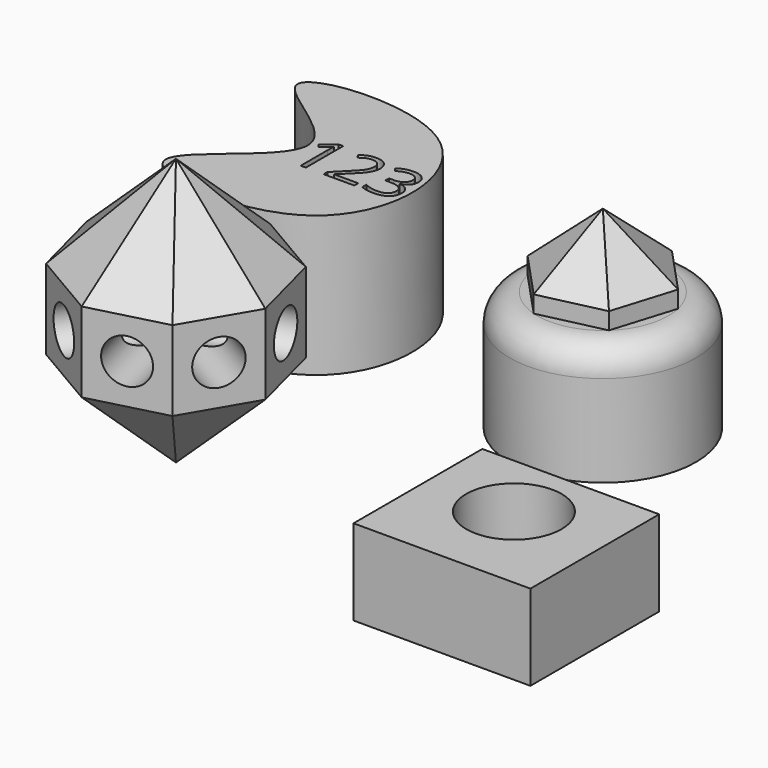
from build123d import *

# Parameters (mm, degrees)
F0_R          = 53.2418373221
F1_DEPTH      = 68.326
F2_R          = 15.9434663659
F3_W          = 92.0383110642
F3_H          = 48.9154662937
F4_DEPTH      = 101.092
F5_R          = 27.2499431861
F6_DEPTH      = 168.402
F8_DEPTH      = 102.87
F9_DEPTH      = 41.91
F11_DEPTH     = 80.264
F12_TEXT_SIZE = 37.3588189379
F13_DEPTH     = 142.748
F14_SIZE      = 32.258
F16_DEPTH     = 152.4
F17_SIZE      = 53.34
F18_SIZE      = 53.34
F19_R         = 12.6996570343
F20_DEPTH     = 120.65
F21_R         = 12.8328111709
F22_DEPTH     = 125.73
F23_R         = 12.8628233785
F24_DEPTH     = 129.032
F25_R         = 12.7876838695
F26_DEPTH     = 111.76


# Not quite as in the source:
# - Text() gives the source's letters only with a copy of the font that has no kerning and outlines rounded to 1/6400 em; it was checked with that copy


with BuildPart() as f1:
    # F0 (on Top) → F1 (new body)
    with BuildSketch(Plane.XY):
        Circle(F0_R)
    extrude(amount=F1_DEPTH)

    # F2
    f2_edges = [f1.edges().sort_by_distance(p)[0] for p in [
        (-53.241837, 0, 68.326),
    ]]
    fillet(f2_edges, radius=F2_R)

    # F7 (on face) → F8 (cut)
    with BuildSketch(Plane.XY.offset(68.326)):
        Polygon((10.9887064491, 35.6429068197), (-25.3733095461, 27.3379523495), (-36.3620159952, -8.3049544702), (-10.9887064491, -35.6429068197), (25.3733095461, -27.3379523495), (36.3620159952, 8.3049544702), align=None)
    extrude(amount=-F8_DEPTH, mode=Mode.SUBTRACT)


with BuildPart() as f4:
    # F3 (on Right) → F4 (new body)
    with BuildSketch(Plane.YZ):
        with Locations((-132.1039460599, -0.1609092578)):
            Rectangle(F3_W, F3_H)
    extrude(amount=F4_DEPTH)

    # F5 (on face) → F6 (cut)
    with BuildSketch(Plane.XY.offset(24.296823889)):
        with Locations((48.7965382636, -124.5229393244)):
            Circle(F5_R)
    extrude(amount=-F6_DEPTH, mode=Mode.SUBTRACT)


with BuildPart() as f9:
    # F7 (on face) → F9 (new body)
    with BuildSketch(Plane.XY.offset(68.326)):
        Polygon((10.9887064491, 35.6429068197), (-25.3733095461, 27.3379523495), (-36.3620159952, -8.3049544702), (-10.9887064491, -35.6429068197), (25.3733095461, -27.3379523495), (36.3620159952, 8.3049544702), align=None)
    extrude(amount=F9_DEPTH)

    # F14
    f14_edges = [f9.edges().sort_by_distance(p)[0] for p in [
        (23.675361, 21.973931, 110.236),
        (-7.192302, 31.49043, 110.236),
        (-30.867663, 9.516499, 110.236),
        (-23.675361, -21.973931, 110.236),
        (7.192302, -31.49043, 110.236),
        (30.867663, -9.516499, 110.236),
    ]]
    chamfer(f14_edges, length=F14_SIZE)


with BuildPart() as f11:
    # F10 (on Top) → F11 (new body)
    with BuildSketch(Plane.XY):
        with BuildLine():
            add(Edge.make_bspline(
                [(-217.9919332266, -39.8857519031), (-217.5246529744, -54.9822862799), (-104.3107234296, -69.2888881971), (-104.8026906793, 77.2163906349), (-264.1316526653, 61.6188569336), (-136.1535719317, 11.8021500487), (-218.4045582352, -26.5549774943), (-217.9919332266, -39.8857519031)],
                knots=[0, 0, 0, 0, 0.209594319, 0.4306655921, 0.6391477534, 0.8149207948, 1, 1, 1, 1], degree=3))
        make_face()
    extrude(amount=F11_DEPTH)

    # F12 (on face) → F13 (cut)
    with BuildSketch(Plane.XY.offset(80.264)):
        with Locations((-177.251736175, -6.9058553999)):
            Text('123', F12_TEXT_SIZE, font='Open Sans', text_align=(TextAlign.LEFT, TextAlign.BOTTOM))
    extrude(amount=-F13_DEPTH, mode=Mode.SUBTRACT)


with BuildPart() as f16:
    # F15 (on Top) → F16 (new body)
    with BuildSketch(Plane.XY):
        Polygon((-93.0019449132, -191.1988758995), (-70.5673117501, -152.9104208992), (-81.7776566789, -109.9727134841), (-120.0661116793, -87.538080321), (-163.0038190943, -98.7484252498), (-185.4384522575, -137.0368802502), (-174.2281073286, -179.9745876652), (-135.9396523283, -202.4092208284), align=None)
    extrude(amount=F16_DEPTH)

    # F17
    f17_edges = [f16.edges().sort_by_distance(p)[0] for p in [
        (-81.784628, -172.054648, 152.4),
        (-76.172484, -131.441567, 152.4),
        (-100.921884, -98.755397, 152.4),
        (-141.534965, -93.143253, 152.4),
        (-174.221136, -117.892653, 152.4),
        (-179.83328, -158.505734, 152.4),
        (-155.08388, -191.191904, 152.4),
        (-114.470799, -196.804048, 152.4),
    ]]
    chamfer(f17_edges, length=F17_SIZE)

    # F18
    f18_edges = [f16.edges().sort_by_distance(p)[0] for p in [
        (-81.784628, -172.054648, 0),
        (-76.172484, -131.441567, 0),
        (-100.921884, -98.755397, 0),
        (-141.534965, -93.143253, 0),
        (-174.221136, -117.892653, 0),
        (-179.83328, -158.505734, 0),
        (-155.08388, -191.191904, 0),
        (-114.470799, -196.804048, 0),
    ]]
    chamfer(f18_edges, length=F18_SIZE)

    # F19 (on face) → F20 (cut)
    with BuildSketch(Plane(origin=(40.7984715071, -156.2657388041, 0), x_dir=(0.9675665955, 0.2526160787, 0), z_dir=(0.2526160787, -0.9675665955, 0))):
        with Locations((-160.4739878859, 76.2)):
            Circle(F19_R)
    extrude(amount=-F20_DEPTH, mode=Mode.SUBTRACT)

    # F21 (on face) → F22 (cut)
    with BuildSketch(Plane(origin=(-123.030954554, -209.9729080854, 0), x_dir=(0.8627994433, -0.5055463586, 0), z_dir=(-0.5055463586, -0.8627994433, 0))):
        with Locations((-37.1499141834, 76.2)):
            Circle(F21_R)
    extrude(amount=-F22_DEPTH, mode=Mode.SUBTRACT)

    # F23 (on face) → F24 (cut)
    with BuildSketch(Plane(origin=(-207.0996679171, -54.0703929429, 0), x_dir=(0.2526160787, -0.9675665955, 0), z_dir=(-0.9675665955, -0.2526160787, 0))):
        with Locations((107.9360754067, 76.2)):
            Circle(F23_R)
    extrude(amount=-F24_DEPTH, mode=Mode.SUBTRACT)

    # F25 (on face) → F26 (cut)
    with BuildSketch(Plane(origin=(-78.2711789466, 45.8620016633, 0), x_dir=(-0.5055463586, -0.8627994433, 0), z_dir=(-0.8627994433, 0.5055463586, 0))):
        with Locations((189.794575893, 76.2)):
            Circle(F25_R)
    extrude(amount=-F26_DEPTH, mode=Mode.SUBTRACT)


solid = Compound([f1.part, f4.part, f9.part, f11.part, f16.part])
